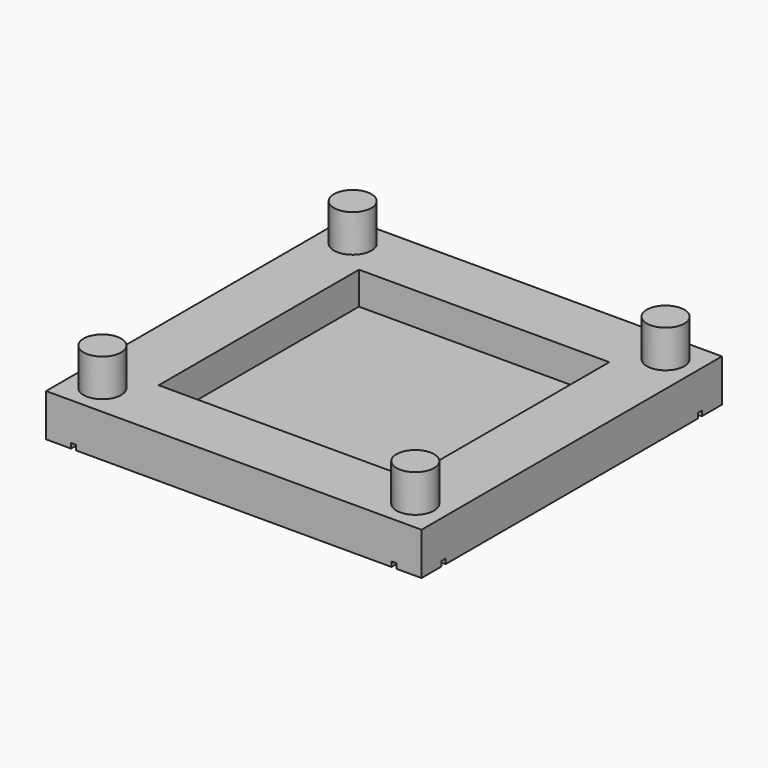
from build123d import *

# Parameters (mm, degrees)
F0_W     = 75
F0_H     = 75
F0_R     = 3.75
F1_DEPTH = 2
F2_DEPTH = 16
F3_W     = 75
F3_H     = 75
F3_R     = 3.75
F3_W_2   = 50
F3_H_2   = 50
F4_DEPTH = 6.5
F5_W     = 1
F5_H     = 1
F6_DEPTH = 1


with BuildPart() as f1:
    # F0 (on Top) → F1 (new body)
    with BuildSketch(Plane.XY):
        Rectangle(F0_W, F0_H)
        with Locations((-31.25, -31.25)):
            Circle(F0_R, mode=Mode.SUBTRACT)
        with Locations((31.25, -31.25)):
            Circle(F0_R, mode=Mode.SUBTRACT)
        with Locations((-31.25, 31.25)):
            Circle(F0_R, mode=Mode.SUBTRACT)
        with Locations((31.25, 31.25)):
            Circle(F0_R, mode=Mode.SUBTRACT)
        with Locations((-31.25, 31.25)):
            Circle(F0_R)
        with Locations((31.25, 31.25)):
            Circle(F0_R)
        with Locations((31.25, -31.25)):
            Circle(F0_R)
        with Locations((-31.25, -31.25)):
            Circle(F0_R)
    extrude(amount=F1_DEPTH)

    # F0 (on Top) → F2 (join)
    with BuildSketch(Plane.XY):
        with Locations((-31.25, -31.25)):
            Circle(F0_R)
        with Locations((31.25, -31.25)):
            Circle(F0_R)
        with Locations((-31.25, 31.25)):
            Circle(F0_R)
        with Locations((31.25, 31.25)):
            Circle(F0_R)
    extrude(amount=F2_DEPTH)

    # F3 (on face) → F4 (join)
    with BuildSketch(Plane.XY.offset(2)):
        Rectangle(F3_W, F3_H)
        with Locations((-31.25, -31.25)):
            Circle(F3_R, mode=Mode.SUBTRACT)
        with Locations((31.25, -31.25)):
            Circle(F3_R, mode=Mode.SUBTRACT)
        with Locations((-31.25, 31.25)):
            Circle(F3_R, mode=Mode.SUBTRACT)
        Rectangle(F3_W_2, F3_H_2, mode=Mode.SUBTRACT)
        with Locations((31.25, 31.25)):
            Circle(F3_R, mode=Mode.SUBTRACT)
    extrude(amount=F4_DEPTH)

    # F5 (on face) → F6 (cut)
    with BuildSketch(Plane.XY):
        with BuildLine():
            Line((-32.5, -34.7855339059), (-32.5, -37.5))
            Line((-32.5, -37.5), (-31.5, -37.5))
            Line((-31.5, -37.5), (-31.5, -34.9916573868))
            ThreePointArc((-31.5, -34.9916573868), (-32.0070480317, -34.9227888964), (-32.5, -34.7855339059))
        make_face()
        with BuildLine():
            Line((-32.5, -32.5), (-32.5, -34.7855339059))
            ThreePointArc((-32.5, -34.7855339059), (-32.0070480317, -34.9227888964), (-31.5, -34.9916573868))
            Line((-31.5, -34.9916573868), (-31.5, -32.5))
            Line((-31.5, -32.5), (-32.5, -32.5))
        make_face()
        with BuildLine():
            Line((31.5, -34.9916573868), (31.5, -37.5))
            Line((31.5, -37.5), (32.5, -37.5))
            Line((32.5, -37.5), (32.5, -34.7855339059))
            ThreePointArc((32.5, -34.7855339059), (32.0070480317, -34.9227888964), (31.5, -34.9916573868))
        make_face()
        with BuildLine():
            Line((-34.7855339059, -32.5), (-32.5, -32.5))
            Line((-32.5, -32.5), (-32.5, -31.5))
            Line((-32.5, -31.5), (-34.9916573868, -31.5))
            ThreePointArc((-34.9916573868, -31.5), (-34.9227888964, -32.0070480317), (-34.7855339059, -32.5))
        make_face()
        with Locations((-32, -32)):
            Rectangle(F5_W, F5_H)
        with BuildLine():
            Line((-37.5, -32.5), (-34.7855339059, -32.5))
            ThreePointArc((-34.7855339059, -32.5), (-34.9227888964, -32.0070480317), (-34.9916573868, -31.5))
            Line((-34.9916573868, -31.5), (-37.5, -31.5))
            Line((-37.5, -31.5), (-37.5, -32.5))
        make_face()
        with BuildLine():
            Line((-31.5, -31.5), (-31.5, -32.5))
            Line((-31.5, -32.5), (-27.7144660941, -32.5))
            ThreePointArc((-27.7144660941, -32.5), (-27.5772111036, -32.0070480317), (-27.5083426132, -31.5))
            Line((-27.5083426132, -31.5), (-31.5, -31.5))
        make_face()
        with BuildLine():
            ThreePointArc((-27.5083426132, -31.5), (-27.5772111036, -32.0070480317), (-27.7144660941, -32.5))
            Line((-27.7144660941, -32.5), (27.7144660941, -32.5))
            ThreePointArc((27.7144660941, -32.5), (27.5772111036, -32.0070480317), (27.5083426132, -31.5))
            Line((27.5083426132, -31.5), (-27.5083426132, -31.5))
        make_face()
        with BuildLine():
            Line((31.5, -32.5), (31.5, -34.9916573868))
            ThreePointArc((31.5, -34.9916573868), (32.0070480317, -34.9227888964), (32.5, -34.7855339059))
            Line((32.5, -34.7855339059), (32.5, -32.5))
            Line((32.5, -32.5), (31.5, -32.5))
        make_face()
        with BuildLine():
            Line((-32.5, -27.7144660941), (-32.5, -31.5))
            Line((-32.5, -31.5), (-31.5, -31.5))
            Line((-31.5, -31.5), (-31.5, -27.5083426132))
            ThreePointArc((-31.5, -27.5083426132), (-32.0070480317, -27.5772111036), (-32.5, -27.7144660941))
        make_face()
        with BuildLine():
            ThreePointArc((27.5083426132, -31.5), (27.5772111036, -32.0070480317), (27.7144660941, -32.5))
            Line((27.7144660941, -32.5), (31.5, -32.5))
            Line((31.5, -32.5), (31.5, -31.5))
            Line((31.5, -31.5), (27.5083426132, -31.5))
        make_face()
        with Locations((32, -32)):
            Rectangle(F5_W, F5_H)
        with BuildLine():
            Line((-32.5, 27.7144660941), (-32.5, -27.7144660941))
            ThreePointArc((-32.5, -27.7144660941), (-32.0070480317, -27.5772111036), (-31.5, -27.5083426132))
            Line((-31.5, -27.5083426132), (-31.5, 27.5083426132))
            ThreePointArc((-31.5, 27.5083426132), (-32.0070480317, 27.5772111036), (-32.5, 27.7144660941))
        make_face()
        with BuildLine():
            Line((-37.5, 32.5), (-37.5, 31.5))
            Line((-37.5, 31.5), (-34.9916573868, 31.5))
            ThreePointArc((-34.9916573868, 31.5), (-34.9227888964, 32.0070480317), (-34.7855339059, 32.5))
            Line((-34.7855339059, 32.5), (-37.5, 32.5))
        make_face()
        with BuildLine():
            Line((32.5, -31.5), (32.5, -32.5))
            Line((32.5, -32.5), (34.7855339059, -32.5))
            ThreePointArc((34.7855339059, -32.5), (34.9227888964, -32.0070480317), (34.9916573868, -31.5))
            Line((34.9916573868, -31.5), (32.5, -31.5))
        make_face()
        with BuildLine():
            ThreePointArc((34.9916573868, -31.5), (34.9227888964, -32.0070480317), (34.7855339059, -32.5))
            Line((34.7855339059, -32.5), (37.5, -32.5))
            Line((37.5, -32.5), (37.5, -31.5))
            Line((37.5, -31.5), (34.9916573868, -31.5))
        make_face()
        with BuildLine():
            Line((31.5, -27.5083426132), (31.5, -31.5))
            Line((31.5, -31.5), (32.5, -31.5))
            Line((32.5, -31.5), (32.5, -27.7144660941))
            ThreePointArc((32.5, -27.7144660941), (32.0070480317, -27.5772111036), (31.5, -27.5083426132))
        make_face()
        with BuildLine():
            Line((-32.5, 31.5), (-32.5, 27.7144660941))
            ThreePointArc((-32.5, 27.7144660941), (-32.0070480317, 27.5772111036), (-31.5, 27.5083426132))
            Line((-31.5, 27.5083426132), (-31.5, 31.5))
            Line((-31.5, 31.5), (-32.5, 31.5))
        make_face()
        with BuildLine():
            ThreePointArc((-34.7855339059, 32.5), (-34.9227888964, 32.0070480317), (-34.9916573868, 31.5))
            Line((-34.9916573868, 31.5), (-32.5, 31.5))
            Line((-32.5, 31.5), (-32.5, 32.5))
            Line((-32.5, 32.5), (-34.7855339059, 32.5))
        make_face()
        with BuildLine():
            Line((31.5, 27.5083426132), (31.5, -27.5083426132))
            ThreePointArc((31.5, -27.5083426132), (32.0070480317, -27.5772111036), (32.5, -27.7144660941))
            Line((32.5, -27.7144660941), (32.5, 27.7144660941))
            ThreePointArc((32.5, 27.7144660941), (32.0070480317, 27.5772111036), (31.5, 27.5083426132))
        make_face()
        with Locations((-32, 32)):
            Rectangle(F5_W, F5_H)
        with BuildLine():
            Line((-31.5, 32.5), (-31.5, 31.5))
            Line((-31.5, 31.5), (-27.5083426132, 31.5))
            ThreePointArc((-27.5083426132, 31.5), (-27.5772111036, 32.0070480317), (-27.7144660941, 32.5))
            Line((-27.7144660941, 32.5), (-31.5, 32.5))
        make_face()
        with BuildLine():
            Line((31.5, 31.5), (31.5, 27.5083426132))
            ThreePointArc((31.5, 27.5083426132), (32.0070480317, 27.5772111036), (32.5, 27.7144660941))
            Line((32.5, 27.7144660941), (32.5, 31.5))
            Line((32.5, 31.5), (31.5, 31.5))
        make_face()
        with BuildLine():
            Line((34.9916573868, 31.5), (37.5, 31.5))
            Line((37.5, 31.5), (37.5, 32.5))
            Line((37.5, 32.5), (34.7855339059, 32.5))
            ThreePointArc((34.7855339059, 32.5), (34.9227888964, 32.0070480317), (34.9916573868, 31.5))
        make_face()
        with BuildLine():
            Line((-32.5, 34.7855339059), (-32.5, 32.5))
            Line((-32.5, 32.5), (-31.5, 32.5))
            Line((-31.5, 32.5), (-31.5, 34.9916573868))
            ThreePointArc((-31.5, 34.9916573868), (-32.0070480317, 34.9227888964), (-32.5, 34.7855339059))
        make_face()
        with BuildLine():
            Line((-32.5, 37.5), (-32.5, 34.7855339059))
            ThreePointArc((-32.5, 34.7855339059), (-32.0070480317, 34.9227888964), (-31.5, 34.9916573868))
            Line((-31.5, 34.9916573868), (-31.5, 37.5))
            Line((-31.5, 37.5), (-32.5, 37.5))
        make_face()
        with BuildLine():
            ThreePointArc((-27.7144660941, 32.5), (-27.5772111036, 32.0070480317), (-27.5083426132, 31.5))
            Line((-27.5083426132, 31.5), (27.5083426132, 31.5))
            ThreePointArc((27.5083426132, 31.5), (27.5772111036, 32.0070480317), (27.7144660941, 32.5))
            Line((27.7144660941, 32.5), (-27.7144660941, 32.5))
        make_face()
        with BuildLine():
            Line((27.5083426132, 31.5), (31.5, 31.5))
            Line((31.5, 31.5), (31.5, 32.5))
            Line((31.5, 32.5), (27.7144660941, 32.5))
            ThreePointArc((27.7144660941, 32.5), (27.5772111036, 32.0070480317), (27.5083426132, 31.5))
        make_face()
        with Locations((32, 32)):
            Rectangle(F5_W, F5_H)
        with BuildLine():
            Line((32.5, 31.5), (34.9916573868, 31.5))
            ThreePointArc((34.9916573868, 31.5), (34.9227888964, 32.0070480317), (34.7855339059, 32.5))
            Line((34.7855339059, 32.5), (32.5, 32.5))
            Line((32.5, 32.5), (32.5, 31.5))
        make_face()
        with BuildLine():
            Line((31.5, 34.9916573868), (31.5, 32.5))
            Line((31.5, 32.5), (32.5, 32.5))
            Line((32.5, 32.5), (32.5, 34.7855339059))
            ThreePointArc((32.5, 34.7855339059), (32.0070480317, 34.9227888964), (31.5, 34.9916573868))
        make_face()
        with BuildLine():
            Line((32.5, 37.5), (31.5, 37.5))
            Line((31.5, 37.5), (31.5, 34.9916573868))
            ThreePointArc((31.5, 34.9916573868), (32.0070480317, 34.9227888964), (32.5, 34.7855339059))
            Line((32.5, 34.7855339059), (32.5, 37.5))
        make_face()
    extrude(amount=F6_DEPTH, mode=Mode.SUBTRACT)


solid = f1.part
